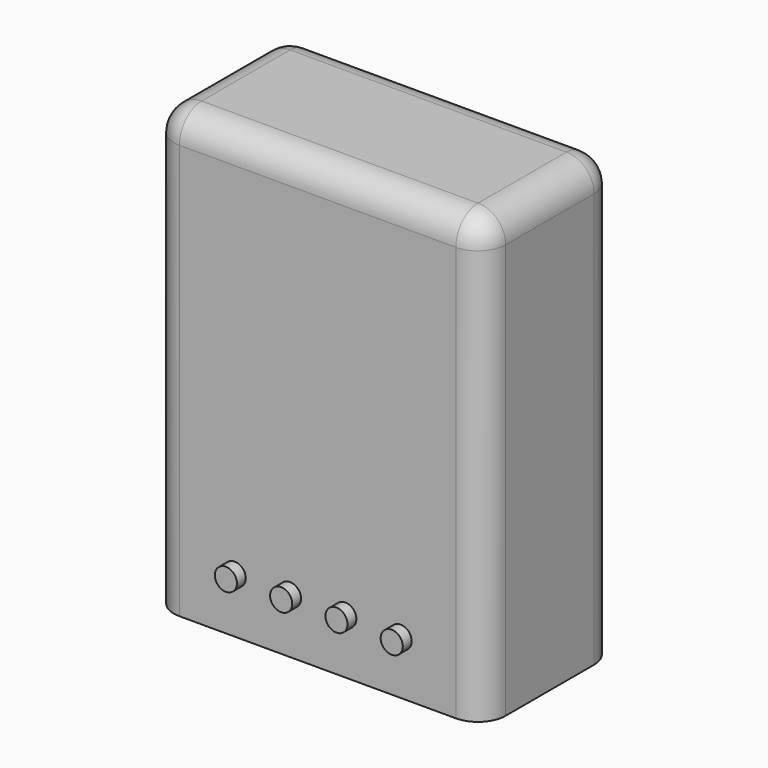
from build123d import *

# Parameters (mm, degrees)
F0_W     = 60
F0_H     = 80
F0_R     = 2
F1_DEPTH = 30
F2_DEPTH = 32
F3_R     = 5


# Not quite as in the source:
# - a feature names something its author has since deleted; it is built from what else it names


with BuildPart() as f1:
    # F0 (on Front) → F1 (new body)
    with BuildSketch(Plane.XZ):
        Rectangle(F0_W, F0_H)
        with Locations((-15, -30.0458669662)):
            Circle(F0_R, mode=Mode.SUBTRACT)
        with Locations((-5, -30.0458669662)):
            Circle(F0_R, mode=Mode.SUBTRACT)
        with Locations((5, -30.0458669662)):
            Circle(F0_R, mode=Mode.SUBTRACT)
        with Locations((15, -30.3212571889)):
            Circle(F0_R, mode=Mode.SUBTRACT)
    extrude(amount=F1_DEPTH)

    # F0 (on Front) → F2 (join)
    with BuildSketch(Plane.XZ):
        with Locations((-15, -30.0458669662)):
            Circle(F0_R)
        with Locations((15, -30.3212571889)):
            Circle(F0_R)
        with Locations((-5, -30.0458669662)):
            Circle(F0_R)
        with Locations((5, -30.0458669662)):
            Circle(F0_R)
    extrude(amount=F2_DEPTH)

    # F3
    f3_edges = [f1.edges().sort_by_distance(p)[0] for p in [
        (0, -30, 40),
        (0, 0, 40),
        (30, -15, 40),
        (-30, -15, 40),
        (-30, -30, 0),
        (30, -30, 0),
        (-30, 0, 0),
        (30, 0, 0),
    ]]
    fillet(f3_edges, radius=F3_R)


solid = f1.part
